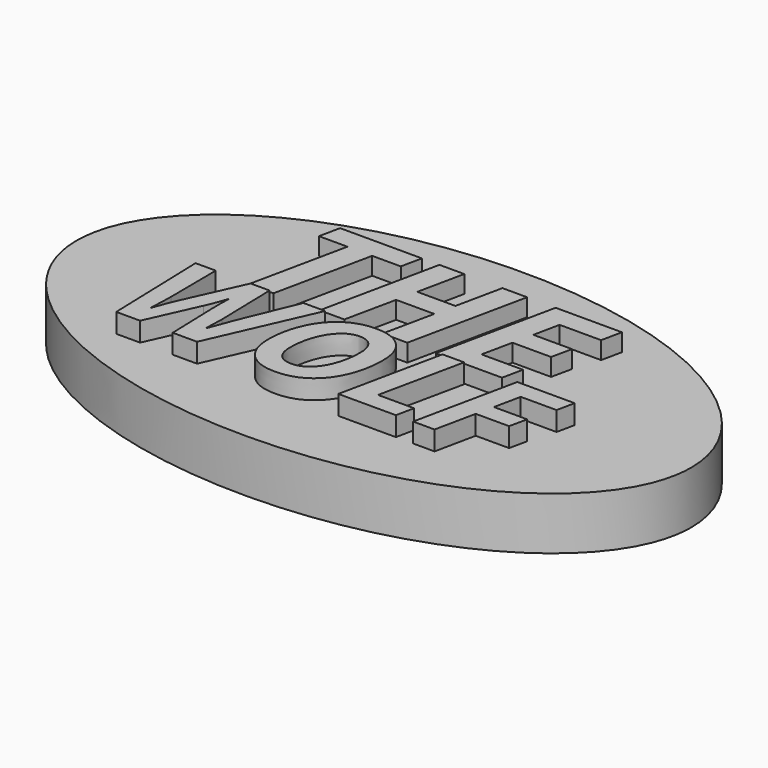
from build123d import *

# Parameters (mm, degrees)
F1_DEPTH     = 7.62
F2_TEXT_SIZE = 24.0014917735
F4_DEPTH     = 2.54
F3_TEXT_SIZE = 20.8772060227
F5_DEPTH     = 2.794


# Not quite as in the source:
# - Text() gives the source's letters only with a copy of the font that has no kerning and outlines rounded to 1/6400 em; it was checked with that copy


with BuildPart() as f1:
    # F0 (on Top) → F1 (new body)
    with BuildSketch(Plane.XY):
        with BuildLine():
            add(Edge.make_bspline(
                [(44.45, 0), (44.45, 43.9940905122), (-22.225, 21.9970452561), (-88.9, 0), (-22.225, -21.9970452561), (44.45, -43.9940905122), (44.45, 0)],
                knots=[0, 0, 0, 2.0943951024, 2.0943951024, 4.1887902048, 4.1887902048, 6.2831853072, 6.2831853072, 6.2831853072], degree=2, weights=[1, 0.5, 1, 0.5, 1, 0.5, 1]))
        make_face()
    extrude(amount=F1_DEPTH)

    # F2 (on face) → F4 (join)
    with BuildSketch(Plane.XY.offset(7.62)):
        with Locations((-22.6694211556, 0)):
            Text('THE', F2_TEXT_SIZE, font='Open Sans', font_style=FontStyle.BOLDITALIC, text_align=(TextAlign.LEFT, TextAlign.BOTTOM))
    extrude(amount=F4_DEPTH)

    # F3 (on face) → F5 (join)
    with BuildSketch(Plane.XY.offset(7.62)):
        with Locations((-29.0323646253, -15.0315883363)):
            Text('WOLF', F3_TEXT_SIZE, font='Open Sans', font_style=FontStyle.BOLDITALIC, text_align=(TextAlign.LEFT, TextAlign.BOTTOM))
    extrude(amount=F5_DEPTH)


solid = f1.part
